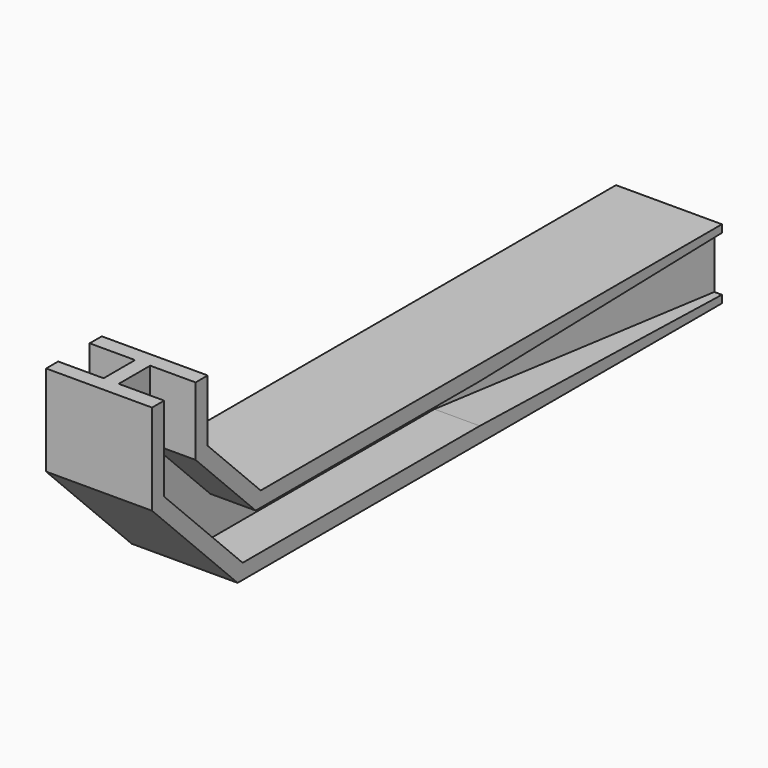
from build123d import *


with BuildPart() as f2:
    # F2: sweep along a path in F1
    with BuildLine(Plane.YZ) as f2_path:
        Line((0, 0), (-254, 0))
        Line((-254, 0), (-343.8025612107, 89.8025612107))
        Line((-343.8025612107, 89.8025612107), (-343.8025612107, 166.0025612107))
    # F0 (on Front) → F2 (sweep)
    with BuildSketch(Plane.XZ):
        Polygon((-88.9, 12.7), (-88.9, 0), (0, 0), (0, 12.7), (-38.1, 12.7), (-38.1, 45.72), (0, 45.72), (0, 58.42), (-88.9, 58.42), (-88.9, 45.72), (-50.8, 45.72), (-50.8, 12.7), align=None)
    sweep(path=f2_path.line, transition=Transition.RIGHT)

    # F2_face (on face) → F5 section 0
    with BuildSketch(Plane(origin=(-44.45, 0, 29.21), x_dir=(-1, 0, 0), z_dir=(0, 1, 0))):
        Polygon((44.45, -16.51), (6.35, -16.51), (6.35, 16.51), (44.45, 16.51), (44.45, 29.21), (-44.45, 29.21), (-44.45, 16.51), (-6.35, 16.51), (-6.35, -16.51), (-44.45, -16.51), (-44.45, -29.21), (44.45, -29.21), align=None)
    # F4 (on offset) → F5 section 1
    with BuildSketch(Plane.XZ.offset(-254)):
        Polygon((-88.9, 0), (0, 0), (0, 6.35), (-6.35, 6.35), (-6.35, 52.07), (0, 52.07), (0, 58.42), (-88.9, 58.42), (-88.9, 52.07), (-82.55, 52.07), (-82.55, 6.35), (-88.9, 6.35), align=None)
    loft()


solid = f2.part
